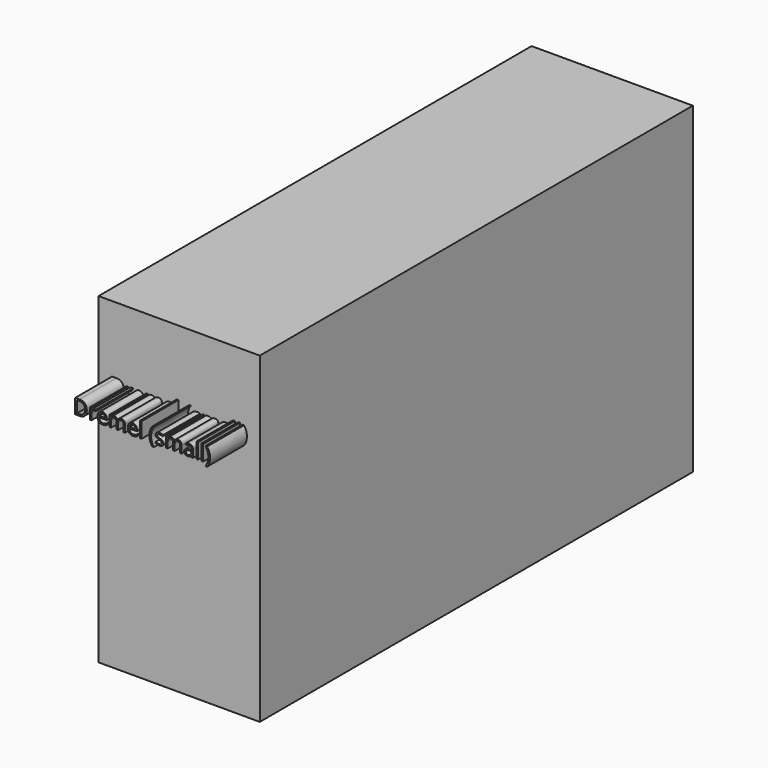
from build123d import *

# Parameters (mm, degrees)
F0_W         = 88.9
F0_H         = 177.8
F1_DEPTH     = 298.45
F2_TEXT_SIZE = 11.2249689269
F3_DEPTH     = 25.4


# Not quite as in the source:
# - Text() gives the source's letters only with a copy of the font that has no kerning and outlines rounded to 1/6400 em; it was checked with that copy


with BuildPart() as f1:
    # F0 (on Front) → F1 (new body)
    with BuildSketch(Plane.XZ):
        Rectangle(F0_W, F0_H)
    extrude(amount=F1_DEPTH)

    # F2 (on face) → F3 (join)
    with BuildSketch(Plane.XZ.offset(298.45)):
        with Locations((-38.1, 44.230034469)):
            Text('Dremel (small)', F2_TEXT_SIZE, font='Open Sans', text_align=(TextAlign.LEFT, TextAlign.BOTTOM))
    extrude(amount=F3_DEPTH)


solid = f1.part
